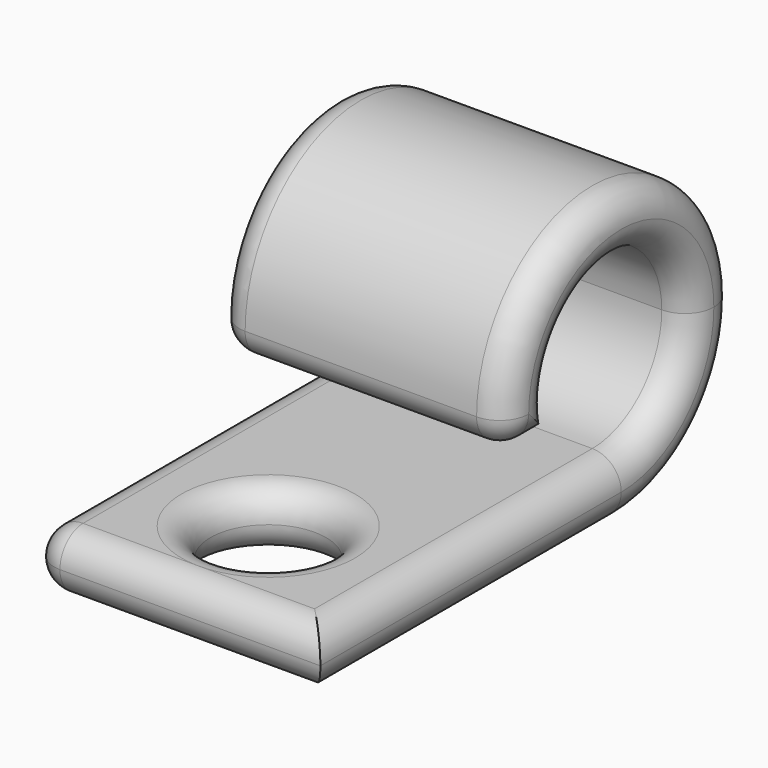
from build123d import *

# Parameters (mm, degrees)
F0_W     = 10
F0_H     = 13
F0_R     = 2
F1_DEPTH = 2
F3_DEPTH = 10
F4_R     = 0.99999


# Not quite as in the source:
# - a fillet or chamfer is up to 0.001 mm smaller than in the source, because OpenCascade refuses the exact size


with BuildPart() as f1:
    # F0 (on Top) → F1 (new body)
    with BuildSketch(Plane.XY):
        with Locations((5, 6.5)):
            Rectangle(F0_W, F0_H)
        with Locations((5, 4)):
            Circle(F0_R, mode=Mode.SUBTRACT)
    extrude(amount=F1_DEPTH)

    # F2 (on Right) → F3 (join)
    with BuildSketch(Plane.YZ):
        with BuildLine():
            ThreePointArc((9, 2), (14.5811388301, 0.2565835097), (18, 5))
            ThreePointArc((18, 5), (12.49745519, 9.974680765), (8.1010205144, 4))
            Line((8.1010205144, 4), (10.1715728753, 4))
            ThreePointArc((10.1715728753, 4), (12.4926940638, 7.956795679), (16, 5))
            ThreePointArc((16, 5), (15.1213203436, 2.8786796564), (13, 2))
            Line((13, 2), (9, 2))
        make_face()
    extrude(amount=F3_DEPTH)

    # F4 (radius 1 in the source; OpenCascade refuses exactly that, so slightly less here)
    f4_edges = [f1.edges().sort_by_distance(p)[0] for p in [
        (0, 6.5, 2),
        (0, 12.492694, 7.956796),
        (0, 0, 1),
        (0, 6.5, 0),
        (0, 16.162278, 8.872983),
        (0, 9.136297, 4),
        (0, 15.12132, 2.87868),
        (10, 12.492694, 7.956796),
        (10, 16.162278, 8.872983),
        (10, 6.5, 2),
        (10, 6.5, 0),
        (5, 8.101021, 4),
        (10, 9.136297, 4),
        (5, 0, 2),
        (5, 0, 0),
        (3, 4, 2),
        (3, 4, 0),
    ]]
    fillet(f4_edges, radius=F4_R)


solid = f1.part
